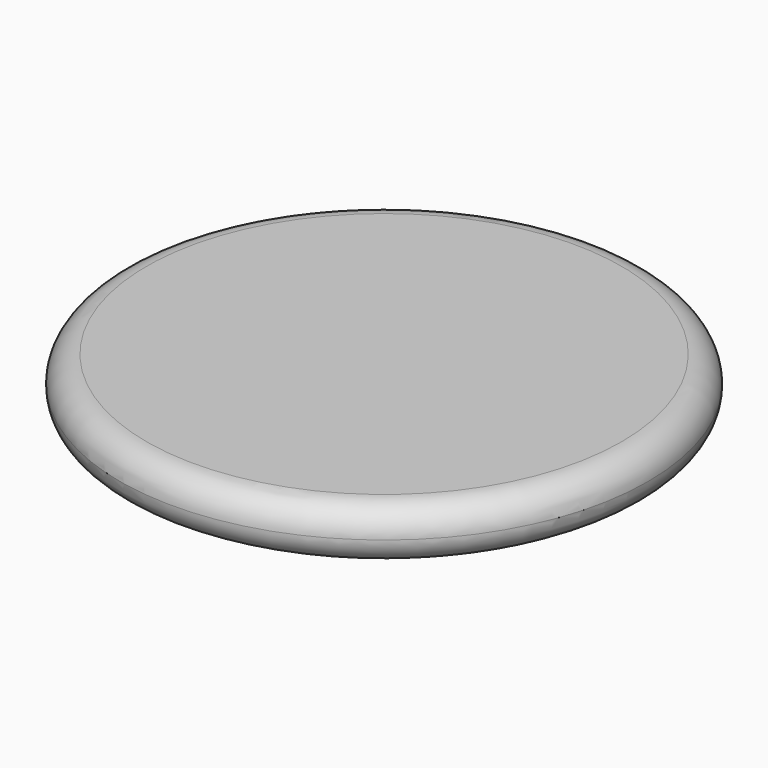
from build123d import *

# Parameters (mm, degrees)
F0_R     = 5
F1_DEPTH = 1
F2_R     = 0.49999


# Not quite as in the source:
# - a fillet or chamfer is up to 0.001 mm smaller than in the source, because OpenCascade refuses the exact size


with BuildPart() as f1:
    # F0 (on Top) → F1 (new body)
    with BuildSketch(Plane.XY):
        Circle(F0_R)
    extrude(amount=F1_DEPTH)

    # F2 (radius 0.5 in the source; OpenCascade refuses exactly that, so slightly less here)
    f2_edges = [f1.edges().sort_by_distance(p)[0] for p in [
        (-5, 0, 1),
        (-5, 0, 0),
    ]]
    fillet(f2_edges, radius=F2_R)


solid = f1.part
